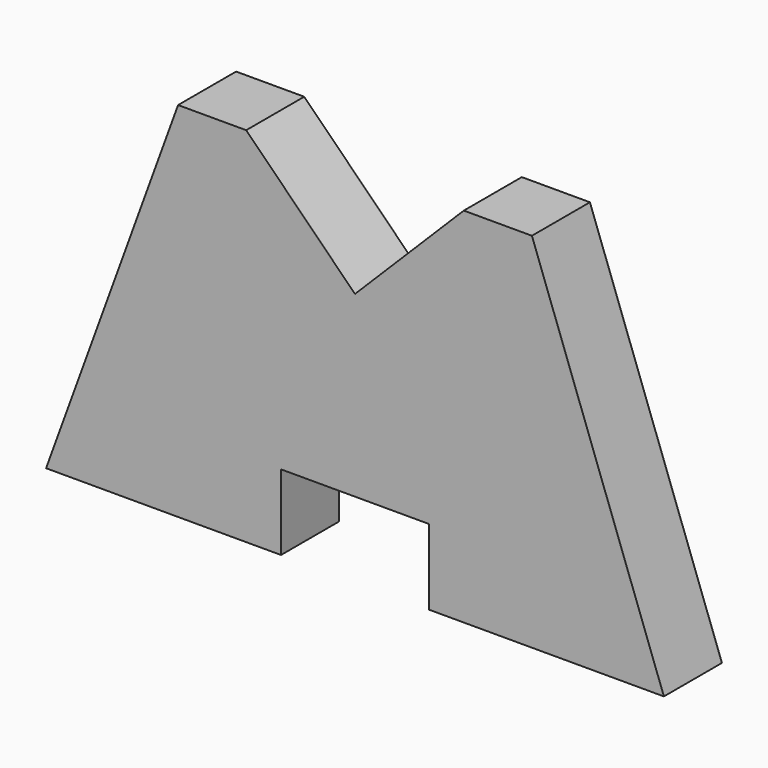
from build123d import *

# Parameters (mm, degrees)
F1_DEPTH = 10


# Not quite as in the source:
# - a feature names something its author has since deleted; it is built from what else it names


with BuildPart() as f1:
    # F0 (on Front) → F1 (new body)
    with BuildSketch(Plane.XZ):
        Polygon((15, 50), (5.6079070177, 50), (-12.5906046956, 0), (19.8, 0), (19.8, 10.4), (40.2, 10.4), (40.2, 0), (72.5906046956, 0), (54.3920929823, 50), (45, 50), (30, 35), align=None)
    extrude(amount=F1_DEPTH)


solid = f1.part
